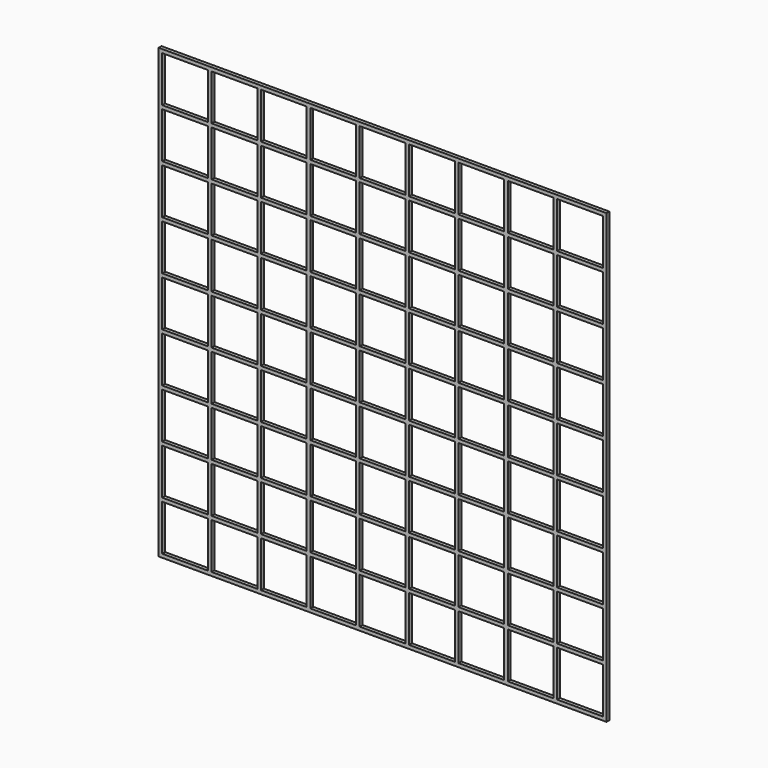
from build123d import *

# Parameters (mm, degrees)
F1_W     = 15.875
F1_H     = 15.875
F1_W_2   = 202.4944444444
F1_H_2   = 202.4944444444
F2_DEPTH = 15.875


# Not quite as in the source:
# - a variable given as a bare number and used for a length is read in inches; the dataset says mm whatever the document's units were


with BuildPart() as f2:
    # F1 (on Front) → F2 (new body)
    with BuildSketch(Plane.XZ):
        with Locations((-982.6625, 982.6625)):
            Rectangle(F1_W, F1_H)
        with Locations((-873.4777777778, 982.6625)):
            Rectangle(F1_W_2, F1_H)
        with Locations((-982.6625, 873.4777777778)):
            Rectangle(F1_W, F1_H_2)
        with Locations((-764.2930555556, 982.6625)):
            Rectangle(F1_W, F1_H)
        with Locations((-982.6625, 764.2930555556)):
            Rectangle(F1_W, F1_H)
        with Locations((-655.1083333333, 982.6625)):
            Rectangle(F1_W_2, F1_H)
        with Locations((-982.6625, 655.1083333333)):
            Rectangle(F1_W, F1_H_2)
        with Locations((-545.9236111111, 982.6625)):
            Rectangle(F1_W, F1_H)
        with Locations((-982.6625, 545.9236111111)):
            Rectangle(F1_W, F1_H)
        with Locations((-436.7388888889, 982.6625)):
            Rectangle(F1_W_2, F1_H)
        with Locations((-982.6625, 436.7388888889)):
            Rectangle(F1_W, F1_H_2)
        with Locations((-327.5541666667, 982.6625)):
            Rectangle(F1_W, F1_H)
        with Locations((-982.6625, 327.5541666667)):
            Rectangle(F1_W, F1_H)
        with Locations((-218.3694444444, 982.6625)):
            Rectangle(F1_W_2, F1_H)
        with Locations((-982.6625, 218.3694444444)):
            Rectangle(F1_W, F1_H_2)
        with Locations((-109.1847222222, 982.6625)):
            Rectangle(F1_W, F1_H)
        with Locations((-982.6625, 109.1847222222)):
            Rectangle(F1_W, F1_H)
        with Locations((0, 982.6625)):
            Rectangle(F1_W_2, F1_H)
        with Locations((-982.6625, 0)):
            Rectangle(F1_W, F1_H_2)
        with Locations((109.1847222222, 982.6625)):
            Rectangle(F1_W, F1_H)
        with Locations((-982.6625, -109.1847222222)):
            Rectangle(F1_W, F1_H)
        with Locations((218.3694444444, 982.6625)):
            Rectangle(F1_W_2, F1_H)
        with Locations((-982.6625, -218.3694444444)):
            Rectangle(F1_W, F1_H_2)
        with Locations((327.5541666667, 982.6625)):
            Rectangle(F1_W, F1_H)
        with Locations((-982.6625, -327.5541666667)):
            Rectangle(F1_W, F1_H)
        with Locations((436.7388888889, 982.6625)):
            Rectangle(F1_W_2, F1_H)
        with Locations((-982.6625, -436.7388888889)):
            Rectangle(F1_W, F1_H_2)
        with Locations((545.9236111111, 982.6625)):
            Rectangle(F1_W, F1_H)
        with Locations((-982.6625, -545.9236111111)):
            Rectangle(F1_W, F1_H)
        with Locations((655.1083333333, 982.6625)):
            Rectangle(F1_W_2, F1_H)
        with Locations((-982.6625, -655.1083333333)):
            Rectangle(F1_W, F1_H_2)
        with Locations((764.2930555556, 982.6625)):
            Rectangle(F1_W, F1_H)
        with Locations((-982.6625, -764.2930555556)):
            Rectangle(F1_W, F1_H)
        with Locations((873.4777777778, 982.6625)):
            Rectangle(F1_W_2, F1_H)
        with Locations((-982.6625, -873.4777777778)):
            Rectangle(F1_W, F1_H_2)
        with Locations((982.6625, 982.6625)):
            Rectangle(F1_W, F1_H)
        with Locations((-982.6625, -982.6625)):
            Rectangle(F1_W, F1_H)
        with Locations((-873.4777777778, -982.6625)):
            Rectangle(F1_W_2, F1_H)
        with Locations((982.6625, 873.4777777778)):
            Rectangle(F1_W, F1_H_2)
        with Locations((-764.2930555556, -982.6625)):
            Rectangle(F1_W, F1_H)
        with Locations((982.6625, 764.2930555556)):
            Rectangle(F1_W, F1_H)
        with Locations((-655.1083333333, -982.6625)):
            Rectangle(F1_W_2, F1_H)
        with Locations((982.6625, 655.1083333333)):
            Rectangle(F1_W, F1_H_2)
        with Locations((-545.9236111111, -982.6625)):
            Rectangle(F1_W, F1_H)
        with Locations((982.6625, 545.9236111111)):
            Rectangle(F1_W, F1_H)
        with Locations((-436.7388888889, -982.6625)):
            Rectangle(F1_W_2, F1_H)
        with Locations((982.6625, 436.7388888889)):
            Rectangle(F1_W, F1_H_2)
        with Locations((-327.5541666667, -982.6625)):
            Rectangle(F1_W, F1_H)
        with Locations((982.6625, 327.5541666667)):
            Rectangle(F1_W, F1_H)
        with Locations((-218.3694444444, -982.6625)):
            Rectangle(F1_W_2, F1_H)
        with Locations((982.6625, 218.3694444444)):
            Rectangle(F1_W, F1_H_2)
        with Locations((-109.1847222222, -982.6625)):
            Rectangle(F1_W, F1_H)
        with Locations((982.6625, 109.1847222222)):
            Rectangle(F1_W, F1_H)
        with Locations((0, -982.6625)):
            Rectangle(F1_W_2, F1_H)
        with Locations((982.6625, 0)):
            Rectangle(F1_W, F1_H_2)
        with Locations((109.1847222222, -982.6625)):
            Rectangle(F1_W, F1_H)
        with Locations((982.6625, -109.1847222222)):
            Rectangle(F1_W, F1_H)
        with Locations((218.3694444444, -982.6625)):
            Rectangle(F1_W_2, F1_H)
        with Locations((982.6625, -218.3694444444)):
            Rectangle(F1_W, F1_H_2)
        with Locations((327.5541666667, -982.6625)):
            Rectangle(F1_W, F1_H)
        with Locations((982.6625, -327.5541666667)):
            Rectangle(F1_W, F1_H)
        with Locations((436.7388888889, -982.6625)):
            Rectangle(F1_W_2, F1_H)
        with Locations((982.6625, -436.7388888889)):
            Rectangle(F1_W, F1_H_2)
        with Locations((545.9236111111, -982.6625)):
            Rectangle(F1_W, F1_H)
        with Locations((982.6625, -545.9236111111)):
            Rectangle(F1_W, F1_H)
        with Locations((655.1083333333, -982.6625)):
            Rectangle(F1_W_2, F1_H)
        with Locations((982.6625, -655.1083333333)):
            Rectangle(F1_W, F1_H_2)
        with Locations((764.2930555556, -982.6625)):
            Rectangle(F1_W, F1_H)
        with Locations((982.6625, -764.2930555556)):
            Rectangle(F1_W, F1_H)
        with Locations((873.4777777778, -982.6625)):
            Rectangle(F1_W_2, F1_H)
        with Locations((982.6625, -873.4777777778)):
            Rectangle(F1_W, F1_H_2)
        with Locations((982.6625, -982.6625)):
            Rectangle(F1_W, F1_H)
        with Locations((-873.4777777778, -109.1847222222)):
            Rectangle(F1_W_2, F1_H)
        with Locations((-873.4777777778, -327.5541666667)):
            Rectangle(F1_W_2, F1_H)
        with Locations((-873.4777777778, -545.9236111111)):
            Rectangle(F1_W_2, F1_H)
        with Locations((-873.4777777778, -764.2930555556)):
            Rectangle(F1_W_2, F1_H)
        with Locations((-764.2930555556, -873.4777777778)):
            Rectangle(F1_W, F1_H_2)
        with Locations((-545.9236111111, -873.4777777778)):
            Rectangle(F1_W, F1_H_2)
        with Locations((-545.9236111111, -655.1083333333)):
            Rectangle(F1_W, F1_H_2)
        with Locations((-655.1083333333, -764.2930555556)):
            Rectangle(F1_W_2, F1_H)
        with Locations((-764.2930555556, -655.1083333333)):
            Rectangle(F1_W, F1_H_2)
        with Locations((-764.2930555556, -436.7388888889)):
            Rectangle(F1_W, F1_H_2)
        with Locations((-764.2930555556, -218.3694444444)):
            Rectangle(F1_W, F1_H_2)
        with Locations((-764.2930555556, 218.3694444444)):
            Rectangle(F1_W, F1_H_2)
        with Locations((-764.2930555556, 436.7388888889)):
            Rectangle(F1_W, F1_H_2)
        with Locations((-873.4777777778, 109.1847222222)):
            Rectangle(F1_W_2, F1_H)
        with Locations((-764.2930555556, 0)):
            Rectangle(F1_W, F1_H_2)
        with Locations((-655.1083333333, 109.1847222222)):
            Rectangle(F1_W_2, F1_H)
        with Locations((-436.7388888889, 109.1847222222)):
            Rectangle(F1_W_2, F1_H)
        with Locations((-545.9236111111, 218.3694444444)):
            Rectangle(F1_W, F1_H_2)
        with Locations((-545.9236111111, 0)):
            Rectangle(F1_W, F1_H_2)
        with Locations((-545.9236111111, 109.1847222222)):
            Rectangle(F1_W, F1_H)
        with Locations((-764.2930555556, 109.1847222222)):
            Rectangle(F1_W, F1_H)
        with Locations((-764.2930555556, -109.1847222222)):
            Rectangle(F1_W, F1_H)
        with Locations((-764.2930555556, 327.5541666667)):
            Rectangle(F1_W, F1_H)
        with Locations((-545.9236111111, 327.5541666667)):
            Rectangle(F1_W, F1_H)
        with Locations((-327.5541666667, 327.5541666667)):
            Rectangle(F1_W, F1_H)
        with Locations((-327.5541666667, 218.3694444444)):
            Rectangle(F1_W, F1_H_2)
        with Locations((-327.5541666667, 109.1847222222)):
            Rectangle(F1_W, F1_H)
        with Locations((-327.5541666667, 0)):
            Rectangle(F1_W, F1_H_2)
        with Locations((-327.5541666667, -109.1847222222)):
            Rectangle(F1_W, F1_H)
        with Locations((-436.7388888889, -109.1847222222)):
            Rectangle(F1_W_2, F1_H)
        with Locations((-545.9236111111, -109.1847222222)):
            Rectangle(F1_W, F1_H)
        with Locations((-655.1083333333, -109.1847222222)):
            Rectangle(F1_W_2, F1_H)
        with Locations((-545.9236111111, -218.3694444444)):
            Rectangle(F1_W, F1_H_2)
        with Locations((-873.4777777778, 327.5541666667)):
            Rectangle(F1_W_2, F1_H)
        with Locations((-655.1083333333, 327.5541666667)):
            Rectangle(F1_W_2, F1_H)
        with Locations((-545.9236111111, 436.7388888889)):
            Rectangle(F1_W, F1_H_2)
        with Locations((-436.7388888889, 327.5541666667)):
            Rectangle(F1_W_2, F1_H)
        with Locations((-327.5541666667, 436.7388888889)):
            Rectangle(F1_W, F1_H_2)
        with Locations((-327.5541666667, 545.9236111111)):
            Rectangle(F1_W, F1_H)
        with Locations((-436.7388888889, 545.9236111111)):
            Rectangle(F1_W_2, F1_H)
        with Locations((-545.9236111111, 545.9236111111)):
            Rectangle(F1_W, F1_H)
        with Locations((-655.1083333333, 545.9236111111)):
            Rectangle(F1_W_2, F1_H)
        with Locations((-873.4777777778, 545.9236111111)):
            Rectangle(F1_W_2, F1_H)
        with Locations((-764.2930555556, 545.9236111111)):
            Rectangle(F1_W, F1_H)
        with Locations((-764.2930555556, 655.1083333333)):
            Rectangle(F1_W, F1_H_2)
        with Locations((-545.9236111111, 655.1083333333)):
            Rectangle(F1_W, F1_H_2)
        with Locations((-327.5541666667, 655.1083333333)):
            Rectangle(F1_W, F1_H_2)
        with Locations((-218.3694444444, 545.9236111111)):
            Rectangle(F1_W_2, F1_H)
        with Locations((-218.3694444444, 327.5541666667)):
            Rectangle(F1_W_2, F1_H)
        with Locations((-218.3694444444, 109.1847222222)):
            Rectangle(F1_W_2, F1_H)
        with Locations((-109.1847222222, 218.3694444444)):
            Rectangle(F1_W, F1_H_2)
        with Locations((-109.1847222222, 109.1847222222)):
            Rectangle(F1_W, F1_H)
        with Locations((-109.1847222222, 327.5541666667)):
            Rectangle(F1_W, F1_H)
        with Locations((-109.1847222222, 545.9236111111)):
            Rectangle(F1_W, F1_H)
        with Locations((-109.1847222222, 764.2930555556)):
            Rectangle(F1_W, F1_H)
        with Locations((-109.1847222222, 655.1083333333)):
            Rectangle(F1_W, F1_H_2)
        with Locations((-218.3694444444, 764.2930555556)):
            Rectangle(F1_W_2, F1_H)
        with Locations((-327.5541666667, 764.2930555556)):
            Rectangle(F1_W, F1_H)
        with Locations((-436.7388888889, 764.2930555556)):
            Rectangle(F1_W_2, F1_H)
        with Locations((-545.9236111111, 764.2930555556)):
            Rectangle(F1_W, F1_H)
        with Locations((-655.1083333333, 764.2930555556)):
            Rectangle(F1_W_2, F1_H)
        with Locations((0, 327.5541666667)):
            Rectangle(F1_W_2, F1_H)
        with Locations((218.3694444444, 327.5541666667)):
            Rectangle(F1_W_2, F1_H)
        with Locations((109.1847222222, 327.5541666667)):
            Rectangle(F1_W, F1_H)
        with Locations((109.1847222222, 218.3694444444)):
            Rectangle(F1_W, F1_H_2)
        with Locations((109.1847222222, 109.1847222222)):
            Rectangle(F1_W, F1_H)
        with Locations((0, 109.1847222222)):
            Rectangle(F1_W_2, F1_H)
        with Locations((109.1847222222, 0)):
            Rectangle(F1_W, F1_H_2)
        with Locations((218.3694444444, 109.1847222222)):
            Rectangle(F1_W_2, F1_H)
        with Locations((327.5541666667, 218.3694444444)):
            Rectangle(F1_W, F1_H_2)
        with Locations((327.5541666667, 109.1847222222)):
            Rectangle(F1_W, F1_H)
        with Locations((327.5541666667, 0)):
            Rectangle(F1_W, F1_H_2)
        with Locations((436.7388888889, 109.1847222222)):
            Rectangle(F1_W_2, F1_H)
        with Locations((545.9236111111, 218.3694444444)):
            Rectangle(F1_W, F1_H_2)
        with Locations((545.9236111111, 109.1847222222)):
            Rectangle(F1_W, F1_H)
        with Locations((545.9236111111, 0)):
            Rectangle(F1_W, F1_H_2)
        with Locations((655.1083333333, 109.1847222222)):
            Rectangle(F1_W_2, F1_H)
        with Locations((655.1083333333, 327.5541666667)):
            Rectangle(F1_W_2, F1_H)
        with Locations((436.7388888889, 327.5541666667)):
            Rectangle(F1_W_2, F1_H)
        with Locations((545.9236111111, 327.5541666667)):
            Rectangle(F1_W, F1_H)
        with Locations((545.9236111111, 436.7388888889)):
            Rectangle(F1_W, F1_H_2)
        with Locations((436.7388888889, 545.9236111111)):
            Rectangle(F1_W_2, F1_H)
        with Locations((-109.1847222222, 436.7388888889)):
            Rectangle(F1_W, F1_H_2)
        with Locations((0, 545.9236111111)):
            Rectangle(F1_W_2, F1_H)
        with Locations((0, 764.2930555556)):
            Rectangle(F1_W_2, F1_H)
        with Locations((109.1847222222, 764.2930555556)):
            Rectangle(F1_W, F1_H)
        with Locations((109.1847222222, 873.4777777778)):
            Rectangle(F1_W, F1_H_2)
        with Locations((109.1847222222, 655.1083333333)):
            Rectangle(F1_W, F1_H_2)
        with Locations((218.3694444444, 545.9236111111)):
            Rectangle(F1_W_2, F1_H)
        with Locations((109.1847222222, 545.9236111111)):
            Rectangle(F1_W, F1_H)
        with Locations((109.1847222222, 436.7388888889)):
            Rectangle(F1_W, F1_H_2)
        with Locations((327.5541666667, 327.5541666667)):
            Rectangle(F1_W, F1_H)
        with Locations((-218.3694444444, -109.1847222222)):
            Rectangle(F1_W_2, F1_H)
        with Locations((-109.1847222222, -109.1847222222)):
            Rectangle(F1_W, F1_H)
        with Locations((-109.1847222222, 0)):
            Rectangle(F1_W, F1_H_2)
        with Locations((0, -109.1847222222)):
            Rectangle(F1_W_2, F1_H)
        with Locations((109.1847222222, -109.1847222222)):
            Rectangle(F1_W, F1_H)
        with Locations((-873.4777777778, 764.2930555556)):
            Rectangle(F1_W_2, F1_H)
        with Locations((-764.2930555556, 764.2930555556)):
            Rectangle(F1_W, F1_H)
        with Locations((-764.2930555556, 873.4777777778)):
            Rectangle(F1_W, F1_H_2)
        with Locations((-545.9236111111, 873.4777777778)):
            Rectangle(F1_W, F1_H_2)
        with Locations((-327.5541666667, 873.4777777778)):
            Rectangle(F1_W, F1_H_2)
        with Locations((218.3694444444, 764.2930555556)):
            Rectangle(F1_W_2, F1_H)
        with Locations((327.5541666667, 873.4777777778)):
            Rectangle(F1_W, F1_H_2)
        with Locations((327.5541666667, 655.1083333333)):
            Rectangle(F1_W, F1_H_2)
        with Locations((327.5541666667, 436.7388888889)):
            Rectangle(F1_W, F1_H_2)
        with Locations((545.9236111111, 655.1083333333)):
            Rectangle(F1_W, F1_H_2)
        with Locations((655.1083333333, 545.9236111111)):
            Rectangle(F1_W_2, F1_H)
        with Locations((545.9236111111, 545.9236111111)):
            Rectangle(F1_W, F1_H)
        with Locations((327.5541666667, 545.9236111111)):
            Rectangle(F1_W, F1_H)
        with Locations((764.2930555556, 545.9236111111)):
            Rectangle(F1_W, F1_H)
        with Locations((764.2930555556, 655.1083333333)):
            Rectangle(F1_W, F1_H_2)
        with Locations((655.1083333333, 764.2930555556)):
            Rectangle(F1_W_2, F1_H)
        with Locations((764.2930555556, 764.2930555556)):
            Rectangle(F1_W, F1_H)
        with Locations((873.4777777778, 109.1847222222)):
            Rectangle(F1_W_2, F1_H)
        with Locations((764.2930555556, 0)):
            Rectangle(F1_W, F1_H_2)
        with Locations((655.1083333333, -109.1847222222)):
            Rectangle(F1_W_2, F1_H)
        with Locations((764.2930555556, -109.1847222222)):
            Rectangle(F1_W, F1_H)
        with Locations((873.4777777778, -109.1847222222)):
            Rectangle(F1_W_2, F1_H)
        with Locations((764.2930555556, -218.3694444444)):
            Rectangle(F1_W, F1_H_2)
        with Locations((436.7388888889, -109.1847222222)):
            Rectangle(F1_W_2, F1_H)
        with Locations((545.9236111111, -109.1847222222)):
            Rectangle(F1_W, F1_H)
        with Locations((545.9236111111, -218.3694444444)):
            Rectangle(F1_W, F1_H_2)
        with Locations((655.1083333333, -327.5541666667)):
            Rectangle(F1_W_2, F1_H)
        with Locations((764.2930555556, -327.5541666667)):
            Rectangle(F1_W, F1_H)
        with Locations((873.4777777778, -327.5541666667)):
            Rectangle(F1_W_2, F1_H)
        with Locations((764.2930555556, -436.7388888889)):
            Rectangle(F1_W, F1_H_2)
        with Locations((764.2930555556, 218.3694444444)):
            Rectangle(F1_W, F1_H_2)
        with Locations((764.2930555556, 436.7388888889)):
            Rectangle(F1_W, F1_H_2)
        with Locations((764.2930555556, 327.5541666667)):
            Rectangle(F1_W, F1_H)
        with Locations((873.4777777778, 327.5541666667)):
            Rectangle(F1_W_2, F1_H)
        with Locations((873.4777777778, 545.9236111111)):
            Rectangle(F1_W_2, F1_H)
        with Locations((873.4777777778, 764.2930555556)):
            Rectangle(F1_W_2, F1_H)
        with Locations((764.2930555556, 873.4777777778)):
            Rectangle(F1_W, F1_H_2)
        with Locations((545.9236111111, 873.4777777778)):
            Rectangle(F1_W, F1_H_2)
        with Locations((545.9236111111, 764.2930555556)):
            Rectangle(F1_W, F1_H)
        with Locations((436.7388888889, 764.2930555556)):
            Rectangle(F1_W_2, F1_H)
        with Locations((327.5541666667, 764.2930555556)):
            Rectangle(F1_W, F1_H)
        with Locations((-109.1847222222, 873.4777777778)):
            Rectangle(F1_W, F1_H_2)
        with Locations((764.2930555556, 109.1847222222)):
            Rectangle(F1_W, F1_H)
        with Locations((327.5541666667, -218.3694444444)):
            Rectangle(F1_W, F1_H_2)
        with Locations((218.3694444444, -109.1847222222)):
            Rectangle(F1_W_2, F1_H)
        with Locations((327.5541666667, -327.5541666667)):
            Rectangle(F1_W, F1_H)
        with Locations((436.7388888889, -327.5541666667)):
            Rectangle(F1_W_2, F1_H)
        with Locations((545.9236111111, -327.5541666667)):
            Rectangle(F1_W, F1_H)
        with Locations((545.9236111111, -436.7388888889)):
            Rectangle(F1_W, F1_H_2)
        with Locations((545.9236111111, -545.9236111111)):
            Rectangle(F1_W, F1_H)
        with Locations((655.1083333333, -545.9236111111)):
            Rectangle(F1_W_2, F1_H)
        with Locations((764.2930555556, -545.9236111111)):
            Rectangle(F1_W, F1_H)
        with Locations((873.4777777778, -545.9236111111)):
            Rectangle(F1_W_2, F1_H)
        with Locations((764.2930555556, -655.1083333333)):
            Rectangle(F1_W, F1_H_2)
        with Locations((764.2930555556, -764.2930555556)):
            Rectangle(F1_W, F1_H)
        with Locations((873.4777777778, -764.2930555556)):
            Rectangle(F1_W_2, F1_H)
        with Locations((764.2930555556, -873.4777777778)):
            Rectangle(F1_W, F1_H_2)
        with Locations((655.1083333333, -764.2930555556)):
            Rectangle(F1_W_2, F1_H)
        with Locations((545.9236111111, -873.4777777778)):
            Rectangle(F1_W, F1_H_2)
        with Locations((545.9236111111, -764.2930555556)):
            Rectangle(F1_W, F1_H)
        with Locations((545.9236111111, -655.1083333333)):
            Rectangle(F1_W, F1_H_2)
        with Locations((436.7388888889, -764.2930555556)):
            Rectangle(F1_W_2, F1_H)
        with Locations((327.5541666667, -764.2930555556)):
            Rectangle(F1_W, F1_H)
        with Locations((327.5541666667, -655.1083333333)):
            Rectangle(F1_W, F1_H_2)
        with Locations((327.5541666667, -545.9236111111)):
            Rectangle(F1_W, F1_H)
        with Locations((436.7388888889, -545.9236111111)):
            Rectangle(F1_W_2, F1_H)
        with Locations((327.5541666667, -436.7388888889)):
            Rectangle(F1_W, F1_H_2)
        with Locations((218.3694444444, -327.5541666667)):
            Rectangle(F1_W_2, F1_H)
        with Locations((109.1847222222, -218.3694444444)):
            Rectangle(F1_W, F1_H_2)
        with Locations((327.5541666667, -109.1847222222)):
            Rectangle(F1_W, F1_H)
        with Locations((327.5541666667, -873.4777777778)):
            Rectangle(F1_W, F1_H_2)
        with Locations((218.3694444444, -764.2930555556)):
            Rectangle(F1_W_2, F1_H)
        with Locations((109.1847222222, -655.1083333333)):
            Rectangle(F1_W, F1_H_2)
        with Locations((109.1847222222, -764.2930555556)):
            Rectangle(F1_W, F1_H)
        with Locations((109.1847222222, -873.4777777778)):
            Rectangle(F1_W, F1_H_2)
        with Locations((0, -764.2930555556)):
            Rectangle(F1_W_2, F1_H)
        with Locations((0, -545.9236111111)):
            Rectangle(F1_W_2, F1_H)
        with Locations((109.1847222222, -545.9236111111)):
            Rectangle(F1_W, F1_H)
        with Locations((218.3694444444, -545.9236111111)):
            Rectangle(F1_W_2, F1_H)
        with Locations((109.1847222222, -436.7388888889)):
            Rectangle(F1_W, F1_H_2)
        with Locations((109.1847222222, -327.5541666667)):
            Rectangle(F1_W, F1_H)
        with Locations((0, -327.5541666667)):
            Rectangle(F1_W_2, F1_H)
        with Locations((-109.1847222222, -218.3694444444)):
            Rectangle(F1_W, F1_H_2)
        with Locations((-109.1847222222, -327.5541666667)):
            Rectangle(F1_W, F1_H)
        with Locations((-109.1847222222, -436.7388888889)):
            Rectangle(F1_W, F1_H_2)
        with Locations((-109.1847222222, -545.9236111111)):
            Rectangle(F1_W, F1_H)
        with Locations((-109.1847222222, -655.1083333333)):
            Rectangle(F1_W, F1_H_2)
        with Locations((-109.1847222222, -764.2930555556)):
            Rectangle(F1_W, F1_H)
        with Locations((-109.1847222222, -873.4777777778)):
            Rectangle(F1_W, F1_H_2)
        with Locations((-218.3694444444, -764.2930555556)):
            Rectangle(F1_W_2, F1_H)
        with Locations((-327.5541666667, -873.4777777778)):
            Rectangle(F1_W, F1_H_2)
        with Locations((-327.5541666667, -764.2930555556)):
            Rectangle(F1_W, F1_H)
        with Locations((-436.7388888889, -764.2930555556)):
            Rectangle(F1_W_2, F1_H)
        with Locations((-327.5541666667, -655.1083333333)):
            Rectangle(F1_W, F1_H_2)
        with Locations((-218.3694444444, -545.9236111111)):
            Rectangle(F1_W_2, F1_H)
        with Locations((-327.5541666667, -545.9236111111)):
            Rectangle(F1_W, F1_H)
        with Locations((-327.5541666667, -436.7388888889)):
            Rectangle(F1_W, F1_H_2)
        with Locations((-218.3694444444, -327.5541666667)):
            Rectangle(F1_W_2, F1_H)
        with Locations((-327.5541666667, -327.5541666667)):
            Rectangle(F1_W, F1_H)
        with Locations((-327.5541666667, -218.3694444444)):
            Rectangle(F1_W, F1_H_2)
        with Locations((-436.7388888889, -327.5541666667)):
            Rectangle(F1_W_2, F1_H)
        with Locations((-545.9236111111, -327.5541666667)):
            Rectangle(F1_W, F1_H)
        with Locations((-545.9236111111, -436.7388888889)):
            Rectangle(F1_W, F1_H_2)
        with Locations((-545.9236111111, -545.9236111111)):
            Rectangle(F1_W, F1_H)
        with Locations((-436.7388888889, -545.9236111111)):
            Rectangle(F1_W_2, F1_H)
        with Locations((-655.1083333333, -545.9236111111)):
            Rectangle(F1_W_2, F1_H)
        with Locations((-655.1083333333, -327.5541666667)):
            Rectangle(F1_W_2, F1_H)
        with Locations((-764.2930555556, -327.5541666667)):
            Rectangle(F1_W, F1_H)
        with Locations((-764.2930555556, -545.9236111111)):
            Rectangle(F1_W, F1_H)
        with Locations((-545.9236111111, -764.2930555556)):
            Rectangle(F1_W, F1_H)
        with Locations((-764.2930555556, -764.2930555556)):
            Rectangle(F1_W, F1_H)
    extrude(amount=F2_DEPTH)


solid = f2.part
